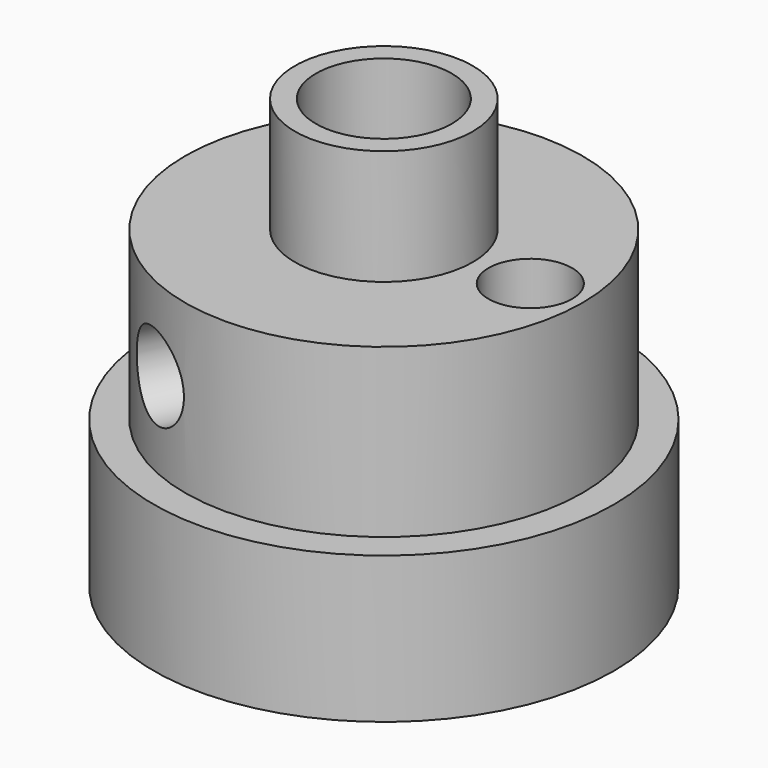
from build123d import *

# Parameters (mm, degrees)
F0_R      = 11
F1_DEPTH  = 7
F2_R      = 9.5
F3_DEPTH  = 8
F4_R      = 4.25
F5_DEPTH  = 5.5
F6_R      = 3.25
F7_DEPTH  = 20.501
F8_R      = 2
F9_DEPTH  = 20.501
F12_R     = 2
F13_DEPTH = 6


# Not quite as in the source:
# - a feature names something its author has since deleted; it is built from what else it names


with BuildPart() as f1:
    # F0 (on Top) → F1 (new body)
    with BuildSketch(Plane.XY):
        Circle(F0_R)
    extrude(amount=F1_DEPTH)

    # F2 (on face) → F3 (join)
    with BuildSketch(Plane.XY.offset(7)):
        Circle(F2_R)
    extrude(amount=F3_DEPTH)

    # F4 (on face) → F5 (join)
    with BuildSketch(Plane.XY.offset(15)):
        Circle(F4_R)
    extrude(amount=F5_DEPTH)

    # F6 (on face) → F7 (cut, through all)
    with BuildSketch(Plane.XY.offset(20.5)):
        Circle(F6_R)
    extrude(amount=-F7_DEPTH, mode=Mode.SUBTRACT)

    # F8 (on face) → F9 (cut, through all)
    with BuildSketch(Plane(origin=(0, 0, 0), x_dir=(1, 0, 0), z_dir=(0, 0, -1))):
        with Locations((7, 0)):
            Circle(F8_R)
    extrude(amount=-F9_DEPTH, mode=Mode.SUBTRACT)

    # F12 (on line) → F13 (cut)
    with BuildSketch(Plane(origin=(-4.0535714286, -8.5917727317, 0), x_dir=(-0.9043971297, 0.4266917293, 0), z_dir=(0.4266917293, 0.9043971297, 0))):
        with Locations((0, 11)):
            Circle(F12_R)
    extrude(amount=F13_DEPTH, mode=Mode.SUBTRACT)


solid = f1.part
